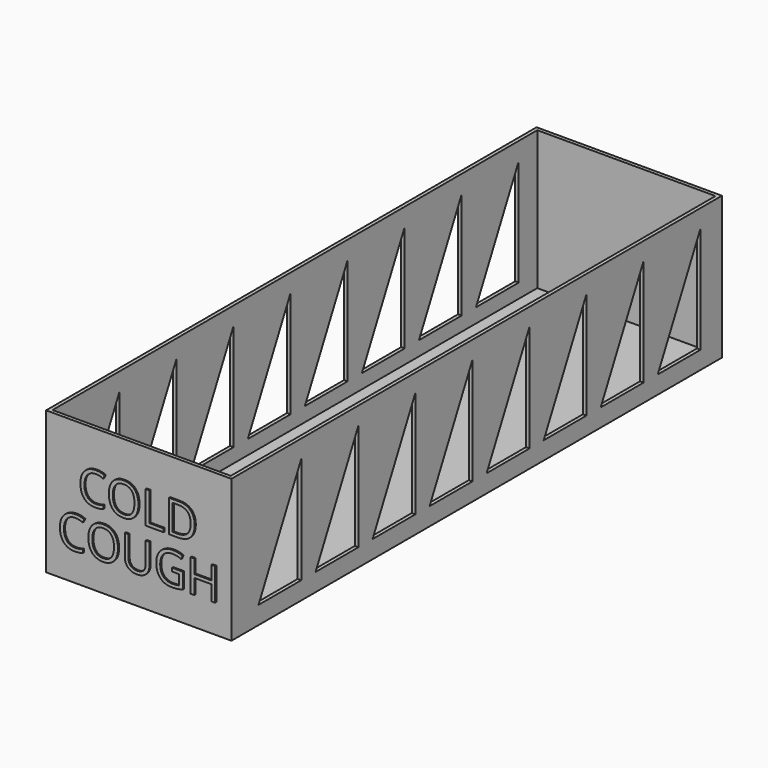
from build123d import *

# Parameters (mm, degrees)
F0_W         = 66.04
F0_H         = 218.44
F0_W_2       = 63.5
F0_H_2       = 215.9
F1_DEPTH     = 1.27
F2_DEPTH     = 50.8
F4_DEPTH     = 76.2
F5_TEXT_SIZE = 16.0513888889
F6_DEPTH     = 0.508


# Not quite as in the source:
# - Text() gives the source's letters only with a copy of the font that has no kerning and outlines rounded to 1/6400 em; it was checked with that copy


with BuildPart() as f1:
    # F0 (on Top) → F1 (new body)
    with BuildSketch(Plane.XY):
        Rectangle(F0_W, F0_H)
        Rectangle(F0_W_2, F0_H_2, mode=Mode.SUBTRACT)
        Rectangle(F0_W_2, F0_H_2)
    extrude(amount=F1_DEPTH)

    # F0 (on Top) → F2 (join)
    with BuildSketch(Plane.XY):
        Rectangle(F0_W, F0_H)
        Rectangle(F0_W_2, F0_H_2, mode=Mode.SUBTRACT)
    extrude(amount=F2_DEPTH)

    # F3 (on face) → F4 (cut)
    with BuildSketch(Plane(origin=(-33.02, 0, 0), x_dir=(0, -1, 0), z_dir=(-1, 0, 0))):
        Polygon((-80.645, 6.35), (-99.695, 44.45), (-99.695, 6.35), align=None)
        Polygon((-74.295, 6.35), (-55.245, 6.35), (-74.295, 44.45), align=None)
        Polygon((-48.895, 6.35), (-29.845, 6.35), (-48.895, 44.45), align=None)
        Polygon((-23.495, 6.35), (-4.445, 6.35), (-23.495, 44.45), align=None)
        Polygon((1.905, 6.35), (20.955, 6.35), (1.905, 44.45), align=None)
        Polygon((27.305, 6.35), (46.355, 6.35), (27.305, 44.45), align=None)
        Polygon((52.705, 6.35), (71.755, 6.35), (52.705, 44.45), align=None)
        Polygon((78.105, 6.35), (97.155, 6.35), (78.105, 44.45), align=None)
    extrude(amount=-F4_DEPTH, mode=Mode.SUBTRACT)

    # F5 (on face) → F6 (join)
    with BuildSketch(Plane.XZ.offset(109.22)):
        with Locations((-21.3608873698, 26.5042591658)):
            Text('COLD', F5_TEXT_SIZE, font='Open Sans', text_align=(TextAlign.LEFT, TextAlign.BOTTOM))
        with Locations((-28.6567452257, 10.3634690271)):
            Text('COUGH', F5_TEXT_SIZE, font='Open Sans', text_align=(TextAlign.LEFT, TextAlign.BOTTOM))
    extrude(amount=F6_DEPTH)


solid = f1.part
